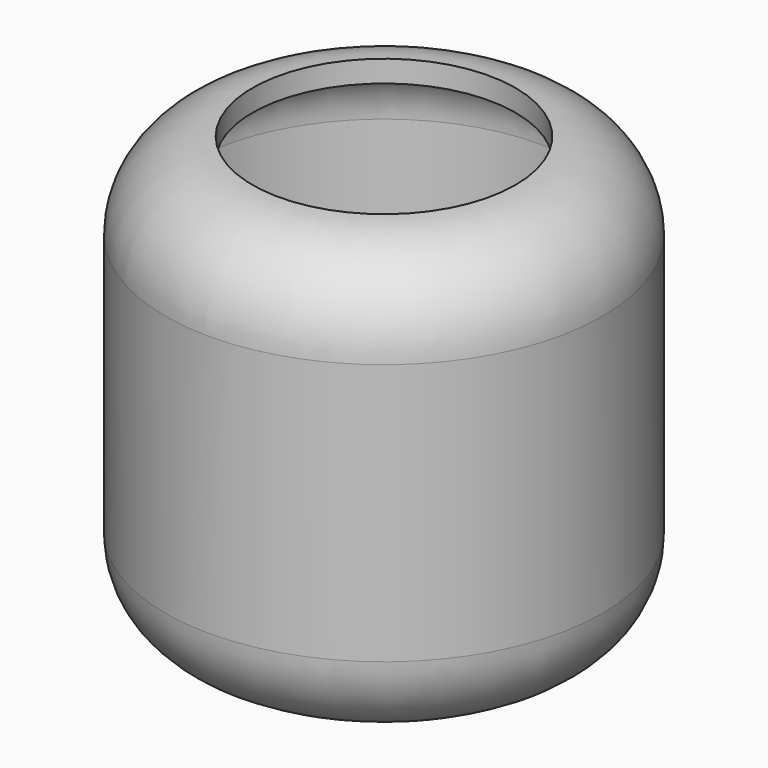
from build123d import *

# Parameters (mm, degrees)
F0_R     = 25.4839572759
F1_DEPTH = 50.8
F2_R     = 10.16
F3_R     = 10.16
F4_T     = -2.54


# Not quite as in the source:
# - a shell that OpenCascade refuses in one call is made with other operations: the cavity is built on its own and cut out


with BuildPart() as f1:
    # F0 (on Top) → F1 (new body)
    with BuildSketch(Plane.XY):
        Circle(F0_R)
    extrude(amount=F1_DEPTH)

    # F2
    f2_edges = [f1.edges().sort_by_distance(p)[0] for p in [
        (-25.483957, 0, 0),
    ]]
    fillet(f2_edges, radius=F2_R)

    # F3
    f3_edges = [f1.edges().sort_by_distance(p)[0] for p in [
        (-25.483957, 0, 50.8),
    ]]
    fillet(f3_edges, radius=F3_R)

    # F4: a shell. OpenCascade refuses it in one call, so the cavity is built on its own and cut out:
    # the body offset inwards by the wall thickness, plus a prism from it out through each open face.
    f4_core = offset(f1.part, amount=F4_T, mode=Mode.PRIVATE)
    f4_exits = [f4_core.faces().sort_by_distance(p)[0] for p in [
        (0, 0, 48.26),
    ]]
    add(f4_core, mode=Mode.SUBTRACT)
    extrude(f4_exits, amount=-F4_T, mode=Mode.SUBTRACT)


solid = f1.part
